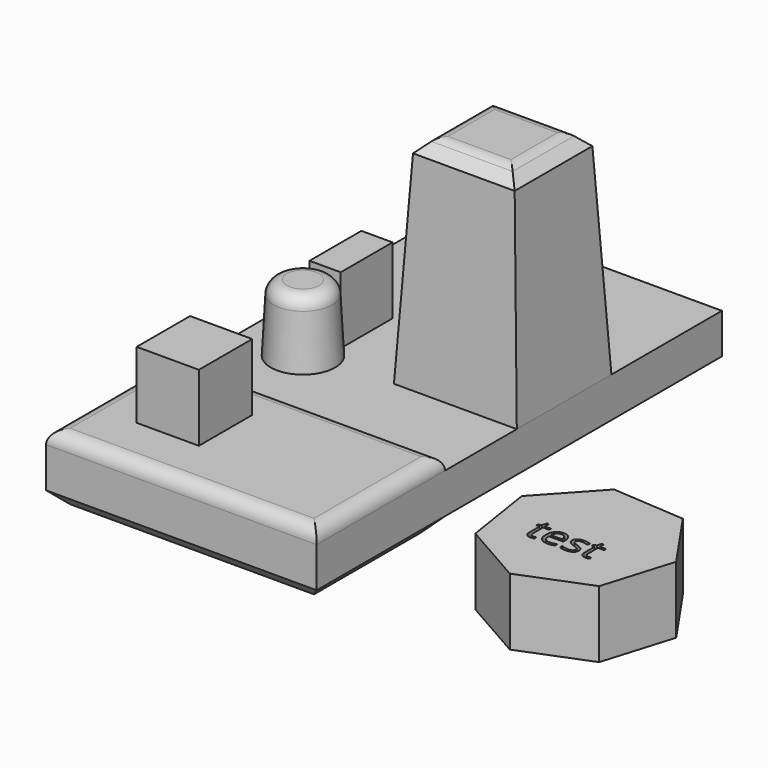
from build123d import *

# Parameters (mm, degrees)
F0_W          = 102.7202121913
F0_H          = 60.888087377
F1_DEPTH      = 25.4
F2_R          = 5.08
F3_SIZE       = 5.08
F4_DEPTH      = 131.39687
F5_W          = 46.6358289123
F5_H          = 44.9039489031
F6_DEPTH      = 81.74897
F6_TAPER      = 3
F7_SIZE       = 5.08
F8_R          = 5.08
F9_R          = 12.2371131237
F10_DEPTH     = 25.4
F10_TAPER     = 3
F11_R         = 5.08
F12_W         = 23.5960744321
F12_H         = 25.3166221082
F13_DEPTH     = 25.4
F15_DEPTH     = 25.4
F16_TEXT_SIZE = 15.0101880232
F17_DEPTH     = 25.401
F18_W         = 11.8279642716
F18_H         = 24.5969687227
F19_DEPTH     = 25.4


# Not quite as in the source:
# - Text() gives the source's letters only with a copy of the font that has no kerning and outlines rounded to 1/6400 em; it was checked with that copy


with BuildPart() as f1:
    # F0 (on Top) → F1 (new body)
    with BuildSketch(Plane.XY):
        with Locations((-51.3601060957, 30.4440436885)):
            Rectangle(F0_W, F0_H)
    extrude(amount=F1_DEPTH)

    # F2
    f2_edges = [f1.edges().sort_by_distance(p)[0] for p in [
        (-51.360106, 0, 25.4),
        (-102.720212, 30.444044, 25.4),
        (-51.360106, 60.888087, 25.4),
        (0, 30.444044, 25.4),
    ]]
    fillet(f2_edges, radius=F2_R)

    # F3
    f3_edges = [f1.edges().sort_by_distance(p)[0] for p in [
        (-51.360106, 0, 0),
        (-102.720212, 30.444044, 0),
        (0, 30.444044, 0),
        (-51.360106, 60.888087, 0),
    ]]
    chamfer(f3_edges, length=F3_SIZE)

    # F4 (add): a face of the model
    f4_faces = [f1.faces().sort_by_distance(p)[0] for p in [
        (-51.3601060957, 60.888087377, 12.7),
    ]]
    extrude(f4_faces, amount=F4_DEPTH)

    # F5 (on face) → F6 (join)
    with BuildSketch(Plane.XY.offset(20.32)):
        with Locations((-23.3179144561, 117.4056306481)):
            Rectangle(F5_W, F5_H)
    extrude(amount=F6_DEPTH, taper=F6_TAPER)

    # F7
    f7_edges = [f1.edges().sort_by_distance(p)[0] for p in [
        (-4.284282, 117.405631, 102.06897),
        (-23.317914, 99.237938, 102.06897),
        (-42.351547, 117.405631, 102.06897),
        (-23.317914, 135.573323, 102.06897),
    ]]
    chamfer(f7_edges, length=F7_SIZE)

    # F8
    f8_edges = [f1.edges().sort_by_distance(p)[0] for p in [
        (-23.317914, 104.317938, 102.06897),
        (-9.364282, 117.405631, 102.06897),
        (-23.317914, 130.493323, 102.06897),
        (-37.271547, 117.405631, 102.06897),
    ]]
    fillet(f8_edges, radius=F8_R)

    # F9 (on face) → F10 (join)
    with BuildSketch(Plane.XY.offset(20.32)):
        with Locations((-78.9942592382, 92.2395065427)):
            Circle(F9_R)
    extrude(amount=F10_DEPTH, taper=F10_TAPER)

    # F11
    f11_edges = [f1.edges().sort_by_distance(p)[0] for p in [
        (-89.900215, 92.239507, 45.72),
    ]]
    fillet(f11_edges, radius=F11_R)

    # F18 (on face) → F19 (join)
    with BuildSketch(Plane.XY.offset(20.32)):
        with Locations((-79.1040006704, 115.1898307441)):
            Rectangle(F18_W, F18_H)
    extrude(amount=F19_DEPTH)


with BuildPart() as f13:
    # F12 (on face) → F13 (new body)
    with BuildSketch(Plane.XY.offset(25.4)):
        with Locations((-72.621146217, 32.7790733427)):
            Rectangle(F12_W, F12_H)
    extrude(amount=F13_DEPTH)


with BuildPart() as f15:
    # F14 (on Top) → F15 (new body)
    with BuildSketch(Plane.XY):
        Polygon((88.1161890245, 23.8969388211), (96.1415567183, 50.4012567198), (80.423381477, 73.2009137564), (52.7977698495, 75.1273031539), (34.0673708512, 54.7298144049), (38.3365569583, 27.3681725703), (62.3905439566, 13.6462520274), align=None)
    extrude(amount=F15_DEPTH)

    # F16 (on face) → F17 (cut, through all)
    with BuildSketch(Plane.XY.offset(25.4)):
        with Locations((49.014993012, 35.7597880065)):
            Text('test', F16_TEXT_SIZE, font='Open Sans', text_align=(TextAlign.LEFT, TextAlign.BOTTOM))
    extrude(amount=-F17_DEPTH, mode=Mode.SUBTRACT)


solid = Compound([f1.part, f13.part, f15.part])
